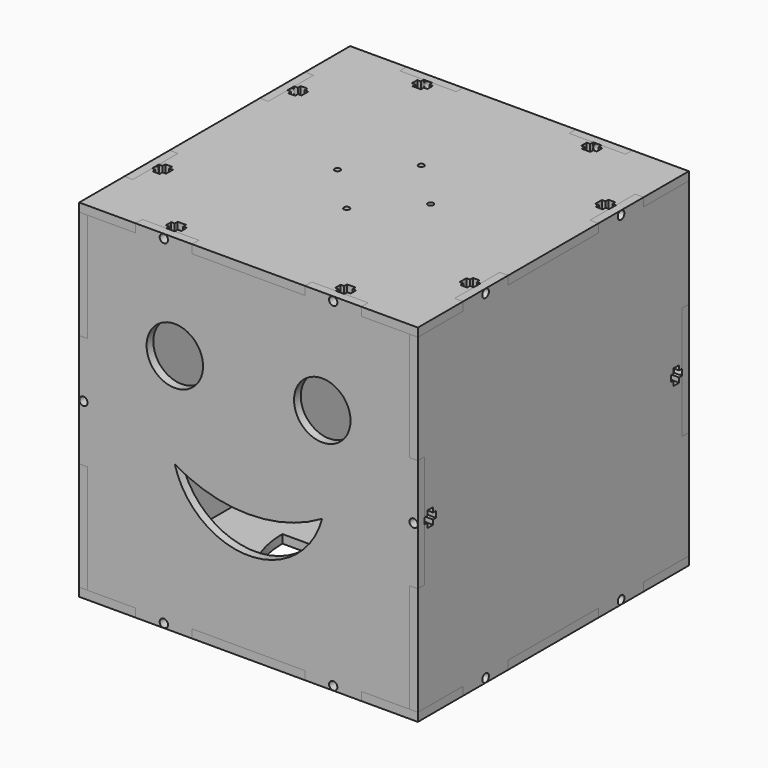
from build123d import *

# Parameters (mm, degrees)
F0_R      = 1
F0_R_2    = 12
F1_DEPTH  = 3
F3_R      = 12
F4_DEPTH  = 3
F7_DEPTH  = 3
F8_R      = 1.475
F9_DEPTH  = 120.001
F12_R     = 1.475
F12_W     = 3
F12_H     = 40
F13_DEPTH = 3
F15_R     = 10
F16_DEPTH = 25
F17_DEPTH = 3


with BuildPart() as f1:
    # F0 (on Top) → F1 (new body)
    with BuildSketch(Plane.XY):
        Polygon((-40, 60), (-60, 60), (-60, 40), (-57, 40), (-57, 31.5), (-55.7, 31.5), (-55.7, 32.75), (-53.3, 32.75), (-53.3, 31.5), (-52, 31.5), (-52, 28.5), (-53.3, 28.5), (-53.3, 27.25), (-55.7, 27.25), (-55.7, 28.5), (-57, 28.5), (-57, 20), (-60, 20), (-60, -20), (-57, -20), (-57, -28.5), (-55.7, -28.5), (-55.7, -27.25), (-53.3, -27.25), (-53.3, -28.5), (-52, -28.5), (-52, -31.5), (-53.3, -31.5), (-53.3, -32.75), (-55.7, -32.75), (-55.7, -31.5), (-57, -31.5), (-57, -40), (-60, -40), (-60, -60), (-40, -60), (-40, -57), (-31.5, -57), (-31.5, -55.7), (-32.75, -55.7), (-32.75, -53.3), (-31.5, -53.3), (-31.5, -52), (-28.5, -52), (-28.5, -53.3), (-27.25, -53.3), (-27.25, -55.7), (-28.5, -55.7), (-28.5, -57), (-20, -57), (-20, -60), (20, -60), (20, -57), (28.5, -57), (28.5, -55.7), (27.25, -55.7), (27.25, -53.3), (28.5, -53.3), (28.5, -52), (31.5, -52), (31.5, -53.3), (32.75, -53.3), (32.75, -55.7), (31.5, -55.7), (31.5, -57), (40, -57), (40, -60), (60, -60), (60, -40), (57, -40), (57, -31.5), (55.7, -31.5), (55.7, -32.75), (53.3, -32.75), (53.3, -31.5), (52, -31.5), (52, -28.5), (53.3, -28.5), (53.3, -27.25), (55.7, -27.25), (55.7, -28.5), (57, -28.5), (57, -20), (60, -20), (60, 20), (57, 20), (57, 28.5), (55.7, 28.5), (55.7, 27.25), (53.3, 27.25), (53.3, 28.5), (52, 28.5), (52, 31.5), (53.3, 31.5), (53.3, 32.75), (55.7, 32.75), (55.7, 31.5), (57, 31.5), (57, 40), (60, 40), (60, 60), (40, 60), (40, 57), (31.5, 57), (31.5, 55.7), (32.75, 55.7), (32.75, 53.3), (31.5, 53.3), (31.5, 52), (28.5, 52), (28.5, 53.3), (27.25, 53.3), (27.25, 55.7), (28.5, 55.7), (28.5, 57), (20, 57), (20, 60), (-20, 60), (-20, 57), (-28.5, 57), (-28.5, 55.7), (-27.25, 55.7), (-27.25, 53.3), (-28.5, 53.3), (-28.5, 52), (-31.5, 52), (-31.5, 53.3), (-32.75, 53.3), (-32.75, 55.7), (-31.5, 55.7), (-31.5, 57), (-40, 57), align=None)
        with BuildLine():
            ThreePointArc((-24, 0), (0, -24), (24, 0))
            Line((24, 0), (36, 0))
            ThreePointArc((36, 0), (0, -36), (-36, 0))
            Line((-36, 0), (-24, 0))
        make_face(mode=Mode.SUBTRACT)
        with Locations((0, -16.5)):
            Circle(F0_R, mode=Mode.SUBTRACT)
        with Locations((-16.5, 0)):
            Circle(F0_R, mode=Mode.SUBTRACT)
        Circle(F0_R_2, mode=Mode.SUBTRACT)
        with Locations((16.5, 0)):
            Circle(F0_R, mode=Mode.SUBTRACT)
        with Locations((0, 16.5)):
            Circle(F0_R, mode=Mode.SUBTRACT)
    extrude(amount=F1_DEPTH)


with BuildPart() as f2_1:
    # F2: copy of F1
    add(f1.part.moved(Location((0, 0, 120))))

    # F3 (on face) → F4 (join)
    with BuildSketch(Plane.XY.offset(123)):
        Circle(F3_R)
    extrude(amount=-F4_DEPTH)

    # F3 (on face) → F17 (join)
    with BuildSketch(Plane.XY.offset(123)):
        with BuildLine():
            Line((-24, 0), (-36, 0))
            ThreePointArc((-36, 0), (0, -36), (36, 0))
            Line((36, 0), (24, 0))
            ThreePointArc((24, 0), (0, -24), (-24, 0))
        make_face()
    extrude(amount=-F17_DEPTH)


with BuildPart() as f7:
    # F6 (on offset) → F7 (new body)
    with BuildSketch(Plane.YZ.offset(60)):
        Polygon((-40, 120), (-60, 120), (-60, 81.5), (-57, 81.5), (-57, 62.5869557261), (-55.7, 62.5869557261), (-55.7, 64.25), (-53.3, 64.25), (-53.3, 62.5869557261), (-52, 62.5869557261), (-52, 60.4130442739), (-53.3, 60.4130442739), (-53.3, 58.75), (-55.7, 58.75), (-55.7, 60.4130442739), (-57, 60.4130442739), (-57, 41.5), (-60, 41.5), (-60, 3), (-40, 3), (-40, 0), (-20, 0), (-20, 3), (20, 3), (20, 0), (40, 0), (40, 3), (60, 3), (60, 41.5), (57, 41.5), (57, 60.4130442739), (55.7, 60.4130442739), (55.7, 58.75), (53.3, 58.75), (53.3, 60.4130442739), (52, 60.4130442739), (52, 62.5869557261), (53.3, 62.5869557261), (53.3, 64.25), (55.7, 64.25), (55.7, 62.5869557261), (57, 62.5869557261), (57, 81.5), (60, 81.5), (60, 120), (40, 120), (40, 123), (20, 123), (20, 120), (-20, 120), (-20, 123), (-40, 123), align=None)
    extrude(amount=-F7_DEPTH)

    # F8 (on face) → F9 (cut, through all)
    with BuildSketch(Plane.YZ.offset(60)):
        with Locations((-30, 121.5)):
            Circle(F8_R)
        with Locations((30, 121.5)):
            Circle(F8_R)
        with Locations((-30, 1.5)):
            Circle(F8_R)
        with Locations((30, 1.5)):
            Circle(F8_R)
    extrude(amount=-F9_DEPTH, mode=Mode.SUBTRACT)


with BuildPart() as f10_1:
    # F10: copy of F7
    add(f7.part.moved(Location((-117, 0, 0))))


with BuildPart() as f13:
    # F12 (on offset) → F13 (new body)
    with BuildSketch(Plane.XZ.offset(-60)):
        Polygon((57, 81.5), (57, 120), (40, 120), (40, 123), (20, 123), (20, 120), (-20, 120), (-20, 123), (-40, 123), (-40, 120), (-57, 120), (-57, 81.5), (-57, 41.5), (-57, 3), (-40, 3), (-40, 0), (-20, 0), (-20, 3), (20, 3), (20, 0), (40, 0), (40, 3), (57, 3), (57, 41.5), (60, 41.5), (60, 81.5), align=None)
        with Locations((-30, 1.5)):
            Circle(F12_R, mode=Mode.SUBTRACT)
        with Locations((30, 1.5)):
            Circle(F12_R, mode=Mode.SUBTRACT)
        with Locations((-30, 121.5)):
            Circle(F12_R, mode=Mode.SUBTRACT)
        with Locations((58.5, 61.5)):
            Circle(F12_R, mode=Mode.SUBTRACT)
        with Locations((30, 121.5)):
            Circle(F12_R, mode=Mode.SUBTRACT)
        with Locations((-58.5, 61.5)):
            Rectangle(F12_W, F12_H)
        with Locations((-58.5, 61.5)):
            Circle(F12_R, mode=Mode.SUBTRACT)
    extrude(amount=F13_DEPTH)


with BuildPart() as f14_1:
    # F14: copy of F13
    add(f13.part.moved(Location((0, -117, 0))))

    # F15 (on face) → F16 (cut)
    with BuildSketch(Plane.XZ.offset(60)):
        with Locations((26.1226147413, 86.1550718546)):
            Circle(F15_R)
        with BuildLine():
            ThreePointArc((26.1226147413, 52.3594357073), (0, 45.2641441349), (-26.1226147413, 52.3594357073))
            ThreePointArc((-26.1226147413, 52.3594357073), (0, 32.3832050372), (26.1226147413, 52.3594357073))
        make_face()
        with Locations((-26.1226147413, 86.1550718546)):
            Circle(F15_R)
    extrude(amount=-F16_DEPTH, mode=Mode.SUBTRACT)


solid = Compound([f1.part, f2_1.part, f7.part, f10_1.part, f13.part, f14_1.part])
